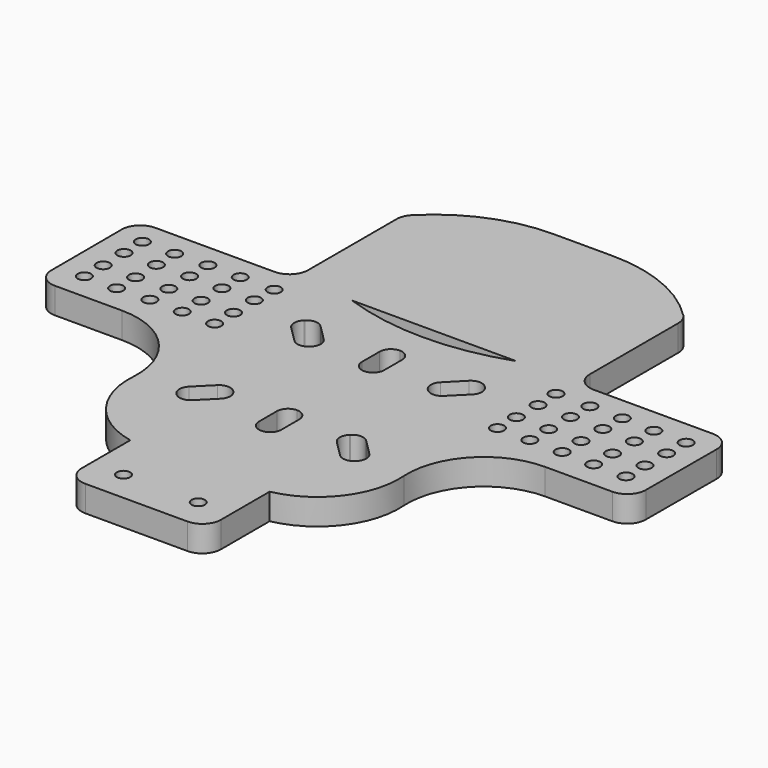
from build123d import *

# Parameters (mm, degrees)
F0_R        = 1.7924715581
F0_W        = 6
F0_H        = 12
F1_DEPTH    = 7
F2_R        = 5
F3_R        = 2.99999
F4_R        = 5
F5_R        = 5
F6_T1_DEPTH = 107.4648585932
F7_R        = 5
F8_R        = 5


# Not quite as in the source:
# - a fillet or chamfer that OpenCascade refuses, or shapes differently, is made with other operations: its cross-section is extruded or revolved along the edge and cut away or added
# - a fillet or chamfer is up to 0.001 mm smaller than in the source, because OpenCascade refuses the exact size


with BuildPart() as f1:
    # F0 (on Top) → F1 (new body)
    with BuildSketch(Plane.XY):
        with BuildLine():
            ThreePointArc((22.0503693582, 33.6896076798), (-0.0002403073, 29.9178496953), (-22.0508499728, 33.6896076798))
            Line((-22.0508499728, 33.6896076798), (-37.8788895905, 33.6896076798))
            Line((-37.8788895905, 33.6896076798), (-80, 33.6896076798))
            Line((-80, 33.6896076798), (-79.9124084099, -0.0643923202))
            Line((-79.9124084099, -0.0643923202), (-56.8817094834, -0.0643923202))
            ThreePointArc((-56.8817094834, -0.0643923202), (-41.9313295872, -6.4745981979), (-36.267593503, -21.72342412))
            ThreePointArc((-36.267593503, -21.72342412), (-31.9176063477, -36.6881030976), (-18.7309216708, -44.9932432158))
            Line((-18.7309216708, -44.9932432158), (-18.7309216708, -66.3649858077))
            Line((-18.7309216708, -66.3649858077), (0, -66.3649858077))
            Line((0, -66.3649858077), (18.7309216708, -66.3649858077))
            Line((18.7309216708, -66.3649858077), (18.7309216708, -44.9932432158))
            ThreePointArc((18.7309216708, -44.9932432158), (31.9176063477, -36.6881030976), (36.267593503, -21.72342412))
            ThreePointArc((36.267593503, -21.72342412), (41.9313295872, -6.4745981979), (56.8817094834, -0.0643923202))
            Line((56.8817094834, -0.0643923202), (79.9124084099, -0.0643923202))
            Line((79.9124084099, -0.0643923202), (80, 33.6896076798))
            Line((80, 33.6896076798), (37.8788895905, 33.6896076798))
            Line((37.8788895905, 33.6896076798), (22.0503693582, 33.6896076798))
        make_face()
        with Locations((-10.05, -58.1420399249)):
            Circle(F0_R, mode=Mode.SUBTRACT)
        with Locations((-72.8230625391, 7.1713337675)):
            Circle(F0_R, mode=Mode.SUBTRACT)
        with Locations((-64.1230625391, 7.1713337675)):
            Circle(F0_R, mode=Mode.SUBTRACT)
        with Locations((-55.4230625391, 7.4549200945)):
            Circle(F0_R, mode=Mode.SUBTRACT)
        with Locations((-46.7230625391, 7.4549200945)):
            Circle(F0_R, mode=Mode.SUBTRACT)
        Polygon((-22.0508499728, -24.7693415731), (-26.4349120161, -20.3852795298), (-17.9496306418, -11.8999981554), (-13.5655685985, -16.2840601989), align=None, mode=Mode.SUBTRACT)
        with Locations((-38.0230625391, 7.4549200945)):
            Circle(F0_R, mode=Mode.SUBTRACT)
        with Locations((10.05, -58.1420399249)):
            Circle(F0_R, mode=Mode.SUBTRACT)
        with Locations((0.059680174, -18.4716808143)):
            Rectangle(F0_W, F0_H, mode=Mode.SUBTRACT)
        Polygon((17.9491500272, -12.0967266704), (26.4344314015, -20.5820080448), (22.0503693582, -24.9660700881), (13.5650879839, -16.4807887139), align=None, mode=Mode.SUBTRACT)
        with Locations((38.0230625391, 7.4549200945)):
            Circle(F0_R, mode=Mode.SUBTRACT)
        with Locations((46.7230625391, 7.4549200945)):
            Circle(F0_R, mode=Mode.SUBTRACT)
        with Locations((55.4230625391, 7.4549200945)):
            Circle(F0_R, mode=Mode.SUBTRACT)
        with Locations((64.1230625391, 7.1713337675)):
            Circle(F0_R, mode=Mode.SUBTRACT)
        with Locations((72.8230625391, 7.1713337675)):
            Circle(F0_R, mode=Mode.SUBTRACT)
        with Locations((-72.8230625391, 13.522426948)):
            Circle(F0_R, mode=Mode.SUBTRACT)
        with Locations((-64.1230625391, 13.522426948)):
            Circle(F0_R, mode=Mode.SUBTRACT)
        with Locations((-72.9498788714, 20.6713337675)):
            Circle(F0_R, mode=Mode.SUBTRACT)
        with Locations((-73.1066465378, 27.022426948)):
            Circle(F0_R, mode=Mode.SUBTRACT)
        with Locations((-64.2498788714, 20.6713337675)):
            Circle(F0_R, mode=Mode.SUBTRACT)
        with Locations((-64.4066465378, 27.022426948)):
            Circle(F0_R, mode=Mode.SUBTRACT)
        with Locations((-55.4230625391, 13.8060132749)):
            Circle(F0_R, mode=Mode.SUBTRACT)
        with Locations((-46.7230625391, 13.8060132749)):
            Circle(F0_R, mode=Mode.SUBTRACT)
        with Locations((-55.5498788714, 20.9549200945)):
            Circle(F0_R, mode=Mode.SUBTRACT)
        with Locations((-55.7066465378, 27.3060132749)):
            Circle(F0_R, mode=Mode.SUBTRACT)
        with Locations((-46.8498788714, 20.9549200945)):
            Circle(F0_R, mode=Mode.SUBTRACT)
        with Locations((-47.0066465378, 27.3060132749)):
            Circle(F0_R, mode=Mode.SUBTRACT)
        with Locations((-38.0230625391, 13.8060132749)):
            Circle(F0_R, mode=Mode.SUBTRACT)
        Polygon((-13.5655685985, 14.0840613981), (-17.9496306418, 9.6999993546), (-26.4349120162, 18.185280729), (-22.0508499728, 22.5693427724), align=None, mode=Mode.SUBTRACT)
        with Locations((-38.1498788714, 20.9549200945)):
            Circle(F0_R, mode=Mode.SUBTRACT)
        with Locations((-37.8788895905, 27.3060132749)):
            Circle(F0_R, mode=Mode.SUBTRACT)
        with Locations((-0.0002403073, 16.1683102548)):
            Rectangle(F0_W, F0_H, mode=Mode.SUBTRACT)
        Polygon((22.0503693582, 22.7077228269), (26.4344314015, 18.1852813744), (17.9491500272, 9.7), (13.5650879839, 14.0840620435), align=None, mode=Mode.SUBTRACT)
        with Locations((38.0230625391, 13.8060132749)):
            Circle(F0_R, mode=Mode.SUBTRACT)
        with Locations((38.1498788714, 20.9549200945)):
            Circle(F0_R, mode=Mode.SUBTRACT)
        with Locations((37.8788895905, 27.3060132749)):
            Circle(F0_R, mode=Mode.SUBTRACT)
        with Locations((46.7230625391, 13.8060132749)):
            Circle(F0_R, mode=Mode.SUBTRACT)
        with Locations((55.4230625391, 13.8060132749)):
            Circle(F0_R, mode=Mode.SUBTRACT)
        with Locations((46.8498788714, 20.9549200945)):
            Circle(F0_R, mode=Mode.SUBTRACT)
        with Locations((47.0066465378, 27.3060132749)):
            Circle(F0_R, mode=Mode.SUBTRACT)
        with Locations((55.5498788714, 20.9549200945)):
            Circle(F0_R, mode=Mode.SUBTRACT)
        with Locations((55.7066465378, 27.3060132749)):
            Circle(F0_R, mode=Mode.SUBTRACT)
        with Locations((64.1230625391, 13.522426948)):
            Circle(F0_R, mode=Mode.SUBTRACT)
        with Locations((72.8230625391, 13.522426948)):
            Circle(F0_R, mode=Mode.SUBTRACT)
        with Locations((64.2498788714, 20.6713337675)):
            Circle(F0_R, mode=Mode.SUBTRACT)
        with Locations((64.4066465378, 27.022426948)):
            Circle(F0_R, mode=Mode.SUBTRACT)
        with Locations((72.9498788714, 20.6713337675)):
            Circle(F0_R, mode=Mode.SUBTRACT)
        with Locations((73.1066465378, 27.022426948)):
            Circle(F0_R, mode=Mode.SUBTRACT)
        Polygon((-37.8788895905, 33.6896076798), (-22.0508499728, 33.6896076798), (0, 33.6896076798), (0.149998191, 33.6896076798), (22.0503693582, 33.6896076798), (37.8788895905, 33.6896076798), (37.8788895905, 70.3556537628), (28.1570665538, 83.6896076798), (-28.1570665538, 83.6896076798), (-37.8788895905, 70.3556537628), align=None)
    extrude(amount=F1_DEPTH)

    # F2
    f2_edges = [f1.edges().sort_by_distance(p)[0] for p in [
        (-80, 33.689608, 3.5),
        (-79.912408, -0.064392, 3.5),
        (-18.730922, -66.364986, 3.5),
        (18.730922, -66.364986, 3.5),
        (79.912408, -0.064392, 3.5),
        (80, 33.689608, 3.5),
    ]]
    fillet(f2_edges, radius=F2_R)

    # F3 (radius 3 in the source; OpenCascade refuses exactly that, so slightly less here)
    f3_edges = [f1.edges().sort_by_distance(p)[0] for p in [
        (-22.05085, 22.569343, 3.5),
        (-13.565569, 14.084061, 3.5),
        (26.434431, 18.185281, 3.5),
        (22.050369, 22.707723, 3.5),
        (2.99976, 22.16831, 3.5),
        (-3.00024, 22.16831, 3.5),
        (-26.434912, 18.185281, 3.5),
        (-3.00024, 10.16831, 3.5),
        (-17.949631, 9.699999, 3.5),
        (17.94915, 9.7, 3.5),
        (13.565088, 14.084062, 3.5),
        (2.99976, 10.16831, 3.5),
        (13.565088, -16.480789, 3.5),
        (-2.94032, -24.471681, 3.5),
        (-2.94032, -12.471681, 3.5),
        (17.94915, -12.096727, 3.5),
        (3.05968, -12.471681, 3.5),
        (26.434431, -20.582008, 3.5),
        (22.050369, -24.96607, 3.5),
        (3.05968, -24.471681, 3.5),
        (-17.949631, -11.899998, 3.5),
        (-26.434912, -20.38528, 3.5),
        (-13.565569, -16.28406, 3.5),
        (-22.05085, -24.769342, 3.5),
    ]]
    fillet(f3_edges, radius=F3_R)

    # F4
    f4_edges = [f1.edges().sort_by_distance(p)[0] for p in [
        (-37.87889, 33.689608, 3.5),
    ]]
    fillet(f4_edges, radius=F4_R)

    # F5
    f5_edges = [f1.edges().sort_by_distance(p)[0] for p in [
        (37.87889, 33.689608, 3.5),
    ]]
    fillet(f5_edges, radius=F5_R)

    # F6: fillet of radius 40 on 2 edges, made by hand

    # F6_s2 → F6_t1 (cut)
    with BuildSketch(Plane.XY.offset(-50.2324292966)):
        with BuildLine():
            ThreePointArc((-8.0640948352, 83.6896076798), (-24.3944064777, 80.2042748926), (-37.8788895905, 70.3556537628))
            Line((-37.8788895905, 70.3556537628), (-28.1570665538, 83.6896076798))
            Line((-28.1570665538, 83.6896076798), (-8.0640948352, 83.6896076798))
        make_face()
        with BuildLine():
            ThreePointArc((37.8788895905, 70.3556537628), (24.3944064777, 80.2042748926), (8.0640948352, 83.6896076798))
            Line((8.0640948352, 83.6896076798), (28.1570665538, 83.6896076798))
            Line((28.1570665538, 83.6896076798), (37.8788895905, 70.3556537628))
        make_face()
    extrude(amount=F6_T1_DEPTH, mode=Mode.SUBTRACT)

    # F7
    f7_edges = [f1.edges().sort_by_distance(p)[0] for p in [
        (-37.87889, 70.355654, 3.5),
    ]]
    fillet(f7_edges, radius=F7_R)

    # F8
    f8_edges = [f1.edges().sort_by_distance(p)[0] for p in [
        (37.87889, 70.355654, 3.5),
    ]]
    fillet(f8_edges, radius=F8_R)


solid = f1.part
